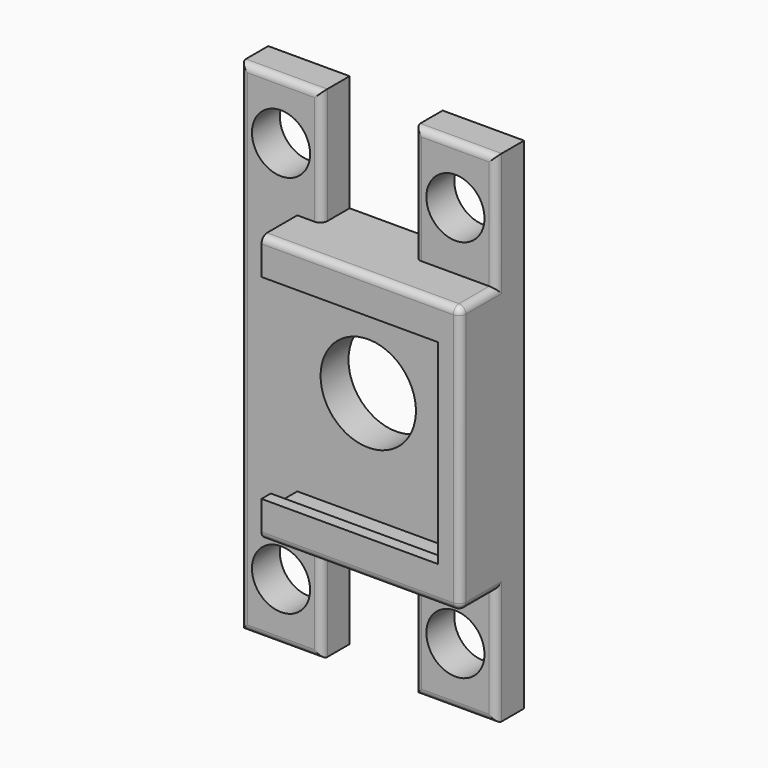
from build123d import *

# Parameters (mm, degrees)
F1_DEPTH      = 3
F2_DEPTH      = 6.85
F6_DEPTH      = 3
F3_W          = 16.2
F3_H          = 1
F7_DEPTH      = 1
F5_W          = 16.2
F5_H          = 1
F8_DEPTH      = 1
F4_W          = 1
F4_H          = 18.8
F9_DEPTH      = 1
F0_W          = 7
F0_H          = 10
F10_DEPTH     = 3
F11_D         = 8.2
F12_D         = 5
F13_R         = 0.6
F14_R         = 0.6
F15_T1_DEPTH  = 18
F15_S5_W      = 0.6
F15_S5_H      = 0.6
F15_T6_DEPTH  = 0.6
F15_S11_W     = 0.6
F15_S11_H     = 0.6
F15_T12_DEPTH = 0.6


# Not quite as in the source:
# - a fillet or chamfer that OpenCascade refuses, or shapes differently, is made with other operations: its cross-section is extruded or revolved along the edge and cut away or added
# - a feature names something its author has since deleted; it is built from what else it names


with BuildPart() as f1:
    # F0 (on Front) → F1 (new body)
    with BuildSketch(Plane.XZ):
        Polygon((0.9, 2.1), (4.9, 2.1), (21.1, 2.1), (21.1, 20.9), (4.9, 20.9), (0.9, 20.9), align=None)
        Polygon((4.9, 2.1), (4.9, 0), (7, 0), (15, 0), (22, 0), (22, 23), (15, 23), (7, 23), (4.9, 23), (4.9, 20.9), (21.1, 20.9), (21.1, 2.1), align=None)
    extrude(amount=F1_DEPTH)

    # F0 (on Front) → F2 (join)
    with BuildSketch(Plane.XZ):
        Polygon((4.9, 2.1), (4.9, 0), (7, 0), (15, 0), (22, 0), (22, 23), (15, 23), (7, 23), (4.9, 23), (4.9, 20.9), (21.1, 20.9), (21.1, 2.1), align=None)
    extrude(amount=F2_DEPTH)

    # F0 (on Front) → F6 (join)
    with BuildSketch(Plane.XZ):
        Polygon((0, 23), (0, 0), (4.9, 0), (4.9, 2.1), (0.9, 2.1), (0.9, 20.9), (4.9, 20.9), (4.9, 23), align=None)
    extrude(amount=F6_DEPTH)

    # F3 (on face) → F7 (join)
    with BuildSketch(Plane(origin=(0, 0, 20.9), x_dir=(1, 0, 0), z_dir=(0, 0, -1))):
        with Locations((13, 6.35)):
            Rectangle(F3_W, F3_H)
    extrude(amount=F7_DEPTH)

    # F5 (on face) → F8 (join)
    with BuildSketch(Plane.XY.offset(2.1)):
        with Locations((13, -6.35)):
            Rectangle(F5_W, F5_H)
    extrude(amount=F8_DEPTH)

    # F4 (on face) → F9 (join)
    with BuildSketch(Plane(origin=(21.1, 0, 0), x_dir=(0, -1, 0), z_dir=(-1, 0, 0))):
        with Locations((6.35, 11.5)):
            Rectangle(F4_W, F4_H)
    extrude(amount=F9_DEPTH)

    # F0 (on Front) → F10 (join)
    with BuildSketch(Plane.XZ):
        with Locations((18.5, 28)):
            Rectangle(F0_W, F0_H)
        with Locations((18.5, -5)):
            Rectangle(F0_W, F0_H)
        Polygon((0, 33), (0, 23), (4.9, 23), (7, 23), (7, 33), align=None)
        Polygon((4.9, 0), (0, 0), (0, -10), (7, -10), (7, 0), align=None)
    extrude(amount=F10_DEPTH)

    # F11 (through all)
    with Locations(Plane(origin=(0, 0, 0), x_dir=(1, 0, 0), z_dir=(0, 1, 0))):
        with Locations((11, -11.5)):
            Hole(F11_D / 2)

    # F12 (through all)
    with Locations(Plane(origin=(0, 0, 0), x_dir=(1, 0, 0), z_dir=(0, 1, 0))):
        with Locations((3.5, -28), (18.5, -28), (3.5, 5), (18.5, 5)):
            Hole(F12_D / 2)

    # F13
    f13_edges = [f1.edges().sort_by_distance(p)[0] for p in [
        (0, -3, 11.5),
        (3.5, -3, -10),
        (7, -3, -5),
        (3.5, -3, 33),
        (7, -3, 28),
    ]]
    fillet(f13_edges, radius=F13_R)

    # F14
    f14_edges = [f1.edges().sort_by_distance(p)[0] for p in [
        (22, -3, -5),
        (18.5, -3, -10),
        (15, -3, -5),
        (22, -4.925, 0),
        (22, -6.85, 11.5),
        (22, -4.925, 23),
        (22, -3, 28),
        (15, -3, 28),
        (18.5, -3, 33),
    ]]
    fillet(f14_edges, radius=F14_R)

    # F15: fillet of radius 0.6 on 2 edges, made by hand

    # F15_s2 → F15_t1 (cut)
    with BuildSketch(Plane.YZ.offset(3.4)):
        with BuildLine():
            ThreePointArc((-6.25, 23), (-6.6742640687, 22.8242640687), (-6.85, 22.4))
            Line((-6.85, 22.4), (-6.85, 23))
            Line((-6.85, 23), (-6.25, 23))
        make_face()
        with BuildLine():
            ThreePointArc((-6.85, 0.6), (-6.6742640687, 0.1757359313), (-6.25, 0))
            Line((-6.25, 0), (-6.85, 0))
            Line((-6.85, 0), (-6.85, 0.6))
        make_face()
    extrude(amount=F15_T1_DEPTH, mode=Mode.SUBTRACT)


with BuildPart() as f15_tool4:
    # F15_s5 → F15_t6 (new body)
    with BuildSketch(Plane.XZ.offset(6.25)):
        with Locations((21.7, 0.3)):
            Rectangle(F15_S5_W, F15_S5_H)
    extrude(amount=F15_T6_DEPTH)

    # F15_s7 → F15_t8 (revolve, cut)
    with BuildSketch(Plane(origin=(21.4, -6.25, 0.6), x_dir=(-0.7071067812, 0, 0.7071067812), z_dir=(0.7071067812, 0, 0.7071067812))):
        with BuildLine():
            ThreePointArc((0, -0.6), (0.6, 0), (0, 0.6))
            Line((0, 0.6), (0, -0.6))
        make_face()
    revolve(axis=Axis((21.4, -6.25, 0.6), (0, -1, 0)), mode=Mode.SUBTRACT)


with BuildPart() as f1_1:
    add(f1.part)

    # F15_t3: cut F15_tool4
    add(f15_tool4.part, mode=Mode.SUBTRACT)


with BuildPart() as f15_tool10:
    # F15_s11 → F15_t12 (new body)
    with BuildSketch(Plane.XY.offset(22.4)):
        with Locations((21.7, -6.55)):
            Rectangle(F15_S11_W, F15_S11_H)
    extrude(amount=F15_T12_DEPTH)

    # F15_s13 → F15_t14 (revolve, cut)
    with BuildSketch(Plane(origin=(21.4, -6.25, 22.4), x_dir=(-0.7071067812, 0.7071067812, 0), z_dir=(0.7071067812, 0.7071067812, 0))):
        with BuildLine():
            ThreePointArc((0, -0.6), (0.6, 0), (0, 0.6))
            Line((0, 0.6), (0, -0.6))
        make_face()
    revolve(axis=Axis((21.4, -6.25, 22.4), (0, 0, 1)), mode=Mode.SUBTRACT)


with BuildPart() as f1_2:
    add(f1_1.part)

    # F15_t9: cut F15_tool10
    add(f15_tool10.part, mode=Mode.SUBTRACT)


solid = f1_2.part
